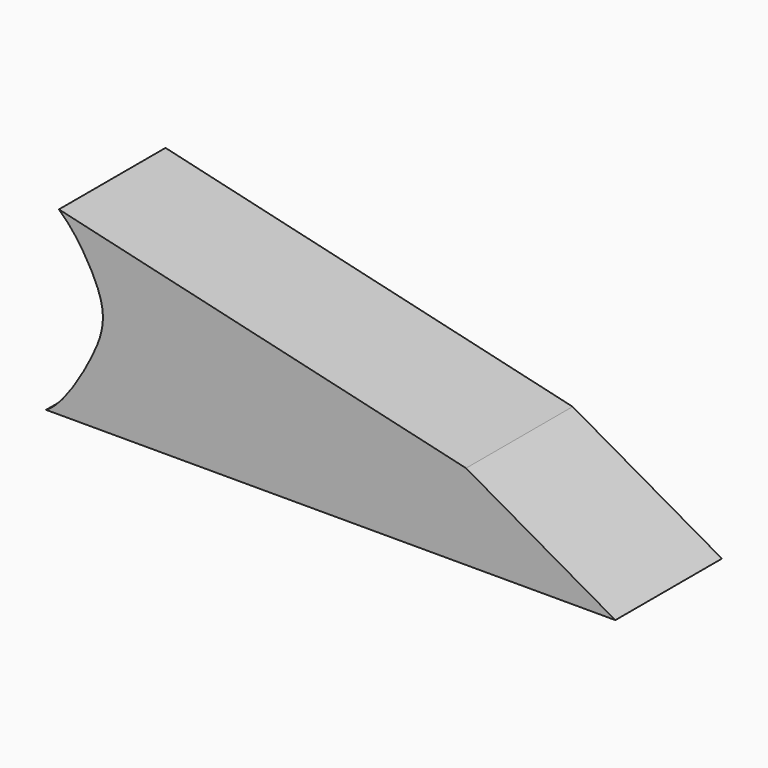
from build123d import *

# Parameters (mm, degrees)
F1_DEPTH = 6.35


with BuildPart() as f1:
    # F0 (on Front) → F1 (new body, symmetric)
    with BuildSketch(Plane.XZ):
        with BuildLine():
            add(Edge.make_bspline(
                [(-5.3486366817, -2.7874862403), (-4.0104451202, -3.9435804676), (-0.5819417824, -9.125605789), (-1.1784647642, -12.8832361111), (-5.0637980722, -19.1799623301), (-6.5756122832, -20.0153414606)],
                knots=[0.0969603728, 0.0969603728, 0.0969603728, 0.0969603728, 0.2285584347, 0.4344976174, 0.602314147, 0.602314147, 0.602314147, 0.602314147], degree=3))
            Line((-6.5756122832, -20.0153414606), (34.656740726, -20.0153416228))
            Line((34.656740726, -20.0153416228), (47.7068386995, -20.0153416742))
            Line((47.7068386995, -20.0153416742), (33.4700680664, -11.8898041731))
            Line((33.4700680664, -11.8898041731), (-5.3486366817, -2.7874862403))
        make_face()
    extrude(amount=F1_DEPTH, both=True)


solid = f1.part
